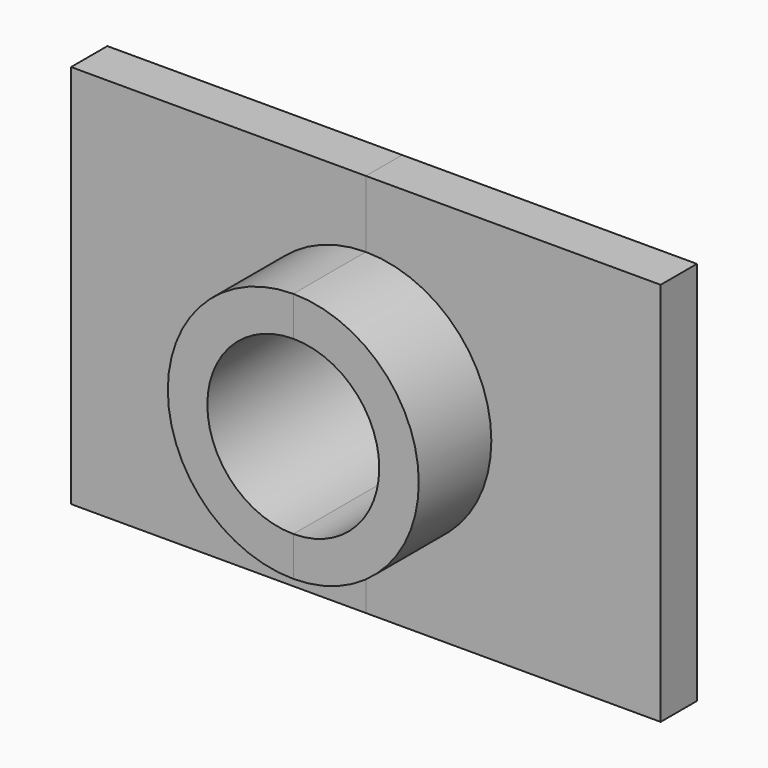
from build123d import *
from build123d import SkipClean  # not in build123d's __all__

# Parameters (mm, degrees)
F1_DEPTH = 25
F3_DEPTH = 5


with BuildPart() as f1:
    # F0 (on Front) → F1 (new body, symmetric)
    with BuildSketch(Plane.XZ):
        with BuildLine():
            Line((0, 27.6668258011), (0, 18.9514327794))
            ThreePointArc((0, 18.9514327794), (18.9514327794, 0), (0, -18.9514327794))
            Line((0, -18.9514327794), (0, -27.6668258011))
            ThreePointArc((0, -27.6668258011), (27.6668258011, 0), (0, 27.6668258011))
        make_face()
    extrude(amount=F1_DEPTH, both=True)

    # F2 (on Front) → F3 (join, symmetric)
    with BuildSketch(Plane.XZ):
        with BuildLine():
            Line((0, 42.4246681583), (0, 27.4246681583))
            ThreePointArc((0, 27.4246681583), (27.4246681583, 0), (0, -27.4246681583))
            Line((0, -27.4246681583), (0, -42.4246681583))
            Line((0, -42.4246681583), (65, -42.4246681583))
            Line((65, -42.4246681583), (65, 42.4246681583))
            Line((65, 42.4246681583), (0, 42.4246681583))
        make_face()
    extrude(amount=F3_DEPTH, both=True)

    # F4: F1 across face


with BuildPart() as f1_1:
    add(f1.part, clean=False)
    with SkipClean():  # cleaning this boolean's faces spoils the solid; the shape is the same uncleaned
        add(f1.part.mirror(Plane(origin=(0, 0, 26.2783197478), x_dir=(0, -1, 0), z_dir=(-1, 0, 0))), clean=False)


solid = f1_1.part
